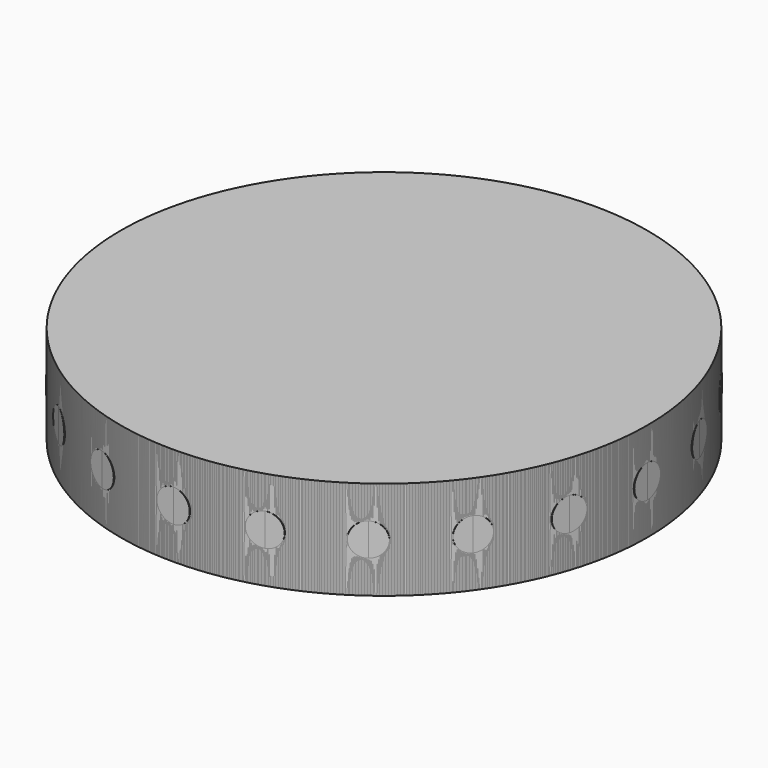
from build123d import *
from build123d import SkipClean  # not in build123d's __all__

# Parameters (mm, degrees)
F0_R     = 25.4
F1_DEPTH = 9.525
F2_R     = 1.585
F3_DEPTH = 5
F4_COUNT = 20


with BuildPart() as f1:
    # F0 (on Top) → F1 (new body)
    with BuildSketch(Plane.XY):
        with Locations((0, -25.4)):
            Circle(F0_R)
    extrude(amount=F1_DEPTH)

    # F2 (on Front) → F3 (join)
    with BuildSketch(Plane.XZ):
        with Locations((0, 4.7625)):
            Circle(F2_R)
    with SkipClean():  # cleaning this boolean's faces spoils the solid; the shape is the same uncleaned
        extrude(amount=F3_DEPTH)


with BuildPart() as f4_1:
    # F4: instance of F1
    add(f1.part.rotate(Axis((0, -25.4, 9.525), (0, 0, 1)), 1 * 360 / F4_COUNT), clean=False)


with BuildPart() as f4_2:
    # F4: instance of F1
    add(f1.part.rotate(Axis((0, -25.4, 9.525), (0, 0, 1)), 2 * 360 / F4_COUNT), clean=False)


with BuildPart() as f4_3:
    # F4: instance of F1
    add(f1.part.rotate(Axis((0, -25.4, 9.525), (0, 0, 1)), 3 * 360 / F4_COUNT), clean=False)


with BuildPart() as f4_4:
    # F4: instance of F1
    add(f1.part.rotate(Axis((0, -25.4, 9.525), (0, 0, 1)), 4 * 360 / F4_COUNT), clean=False)


with BuildPart() as f4_5:
    # F4: instance of F1
    add(f1.part.rotate(Axis((0, -25.4, 9.525), (0, 0, 1)), 5 * 360 / F4_COUNT), clean=False)


with BuildPart() as f4_6:
    # F4: instance of F1
    add(f1.part.rotate(Axis((0, -25.4, 9.525), (0, 0, 1)), 6 * 360 / F4_COUNT), clean=False)


with BuildPart() as f4_7:
    # F4: instance of F1
    add(f1.part.rotate(Axis((0, -25.4, 9.525), (0, 0, 1)), 7 * 360 / F4_COUNT), clean=False)


with BuildPart() as f4_8:
    # F4: instance of F1
    add(f1.part.rotate(Axis((0, -25.4, 9.525), (0, 0, 1)), 8 * 360 / F4_COUNT), clean=False)


with BuildPart() as f4_9:
    # F4: instance of F1
    add(f1.part.rotate(Axis((0, -25.4, 9.525), (0, 0, 1)), 9 * 360 / F4_COUNT), clean=False)


with BuildPart() as f4_10:
    # F4: instance of F1
    add(f1.part.rotate(Axis((0, -25.4, 9.525), (0, 0, 1)), 10 * 360 / F4_COUNT), clean=False)


with BuildPart() as f4_11:
    # F4: instance of F1
    add(f1.part.rotate(Axis((0, -25.4, 9.525), (0, 0, 1)), 11 * 360 / F4_COUNT), clean=False)


with BuildPart() as f4_12:
    # F4: instance of F1
    add(f1.part.rotate(Axis((0, -25.4, 9.525), (0, 0, 1)), 12 * 360 / F4_COUNT), clean=False)


with BuildPart() as f4_13:
    # F4: instance of F1
    add(f1.part.rotate(Axis((0, -25.4, 9.525), (0, 0, 1)), 13 * 360 / F4_COUNT), clean=False)


with BuildPart() as f4_14:
    # F4: instance of F1
    add(f1.part.rotate(Axis((0, -25.4, 9.525), (0, 0, 1)), 14 * 360 / F4_COUNT), clean=False)


with BuildPart() as f4_15:
    # F4: instance of F1
    add(f1.part.rotate(Axis((0, -25.4, 9.525), (0, 0, 1)), 15 * 360 / F4_COUNT), clean=False)


with BuildPart() as f4_16:
    # F4: instance of F1
    add(f1.part.rotate(Axis((0, -25.4, 9.525), (0, 0, 1)), 16 * 360 / F4_COUNT), clean=False)


with BuildPart() as f4_17:
    # F4: instance of F1
    add(f1.part.rotate(Axis((0, -25.4, 9.525), (0, 0, 1)), 17 * 360 / F4_COUNT), clean=False)


with BuildPart() as f4_18:
    # F4: instance of F1
    add(f1.part.rotate(Axis((0, -25.4, 9.525), (0, 0, 1)), 18 * 360 / F4_COUNT), clean=False)


with BuildPart() as f4_19:
    # F4: instance of F1
    add(f1.part.rotate(Axis((0, -25.4, 9.525), (0, 0, 1)), 19 * 360 / F4_COUNT), clean=False)


solid = Compound([f1.part, f4_1.part, f4_2.part, f4_3.part, f4_4.part, f4_5.part, f4_6.part, f4_7.part, f4_8.part, f4_9.part, f4_10.part, f4_11.part, f4_12.part, f4_13.part, f4_14.part, f4_15.part, f4_16.part, f4_17.part, f4_18.part, f4_19.part])
